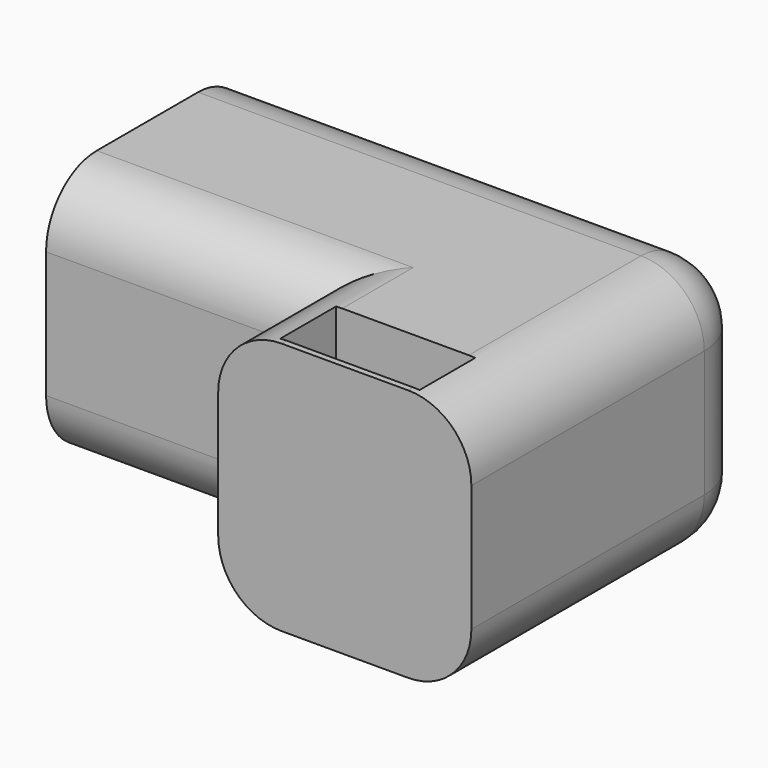
from build123d import *

# Parameters (mm, degrees)
F1_DEPTH     = 20
F2_DEPTH     = 5
F3_R         = 6.25
F4_DEPTH     = 10
F5_R         = 1.4
F6_DEPTH     = 3.9098179487
F7_T1_DEPTH  = 47.5
F7_T3_DEPTH  = 32.5
F7_T5_DEPTH  = 20.5
F7_T7_DEPTH  = 35.5
F7_T9_DEPTH  = 10
F7_S13_W     = 5
F7_S13_H     = 5
F7_T14_DEPTH = 5
F7_S19_W     = 5
F7_S19_H     = 5
F7_T20_DEPTH = 5
F7_T27_DEPTH = 45
F7_T31_DEPTH = 33
F7_T38_DEPTH = 45
F7_T42_DEPTH = 33


# Not quite as in the source:
# - a fillet or chamfer that OpenCascade refuses, or shapes differently, is made with other operations: its cross-section is extruded or revolved along the edge and cut away or added


with BuildPart() as f1:
    # F0 (on Top) → F1 (new body)
    with BuildSketch(Plane.XY):
        Polygon((0, 10), (0, 0), (0, -10), (20, -10), (20, -18), (40, -18), (40, 10), align=None)
        Polygon((35.5, -12), (35.5, -17.5), (30, -17.5), (24.5, -17.5), (24.5, -12), align=None, mode=Mode.SUBTRACT)
    extrude(amount=F1_DEPTH)

    # F0 (on Top) → F2 (join)
    with BuildSketch(Plane.XY):
        Polygon((30, -17.5), (35.5, -17.5), (35.5, -12), (24.5, -12), (24.5, -17.5), align=None)
    extrude(amount=F2_DEPTH)

    # F3 (on face) → F4 (cut)
    with BuildSketch(Plane(origin=(0, 0, 0), x_dir=(0, -1, 0), z_dir=(-1, 0, 0))):
        with Locations((0, 10)):
            Circle(F3_R)
    extrude(amount=-F4_DEPTH, mode=Mode.SUBTRACT)

    # F5 (on face) → F6 (cut, through all)
    with BuildSketch(Plane(origin=(0, 10, 0), x_dir=(-1, 0, 0), z_dir=(0, 1, 0))):
        with Locations((-5, 10)):
            Circle(F5_R)
    extrude(amount=-F6_DEPTH, mode=Mode.SUBTRACT)

    # F7: fillet of radius 5 on 9 edges, made by hand

    # F7_s2 → F7_t1 (cut)
    with BuildSketch(Plane.YZ.offset(-12.5)):
        with BuildLine():
            ThreePointArc((10, 15), (8.5355339059, 18.5355339059), (5, 20))
            Line((5, 20), (10, 20))
            Line((10, 20), (10, 15))
        make_face()
        with BuildLine():
            ThreePointArc((10, 5), (8.5355339059, 1.4644660941), (5, 0))
            Line((5, 0), (10, 0))
            Line((10, 0), (10, 5))
        make_face()
    extrude(amount=F7_T1_DEPTH, mode=Mode.SUBTRACT)

    # F7_s4 → F7_t3 (cut)
    with BuildSketch(Plane.YZ.offset(-12.5)):
        with BuildLine():
            ThreePointArc((-5, 20), (-8.5355339059, 18.5355339059), (-10, 15))
            Line((-10, 15), (-10, 20))
            Line((-10, 20), (-5, 20))
        make_face()
        with BuildLine():
            ThreePointArc((-5, 0), (-8.5355339059, 1.4644660941), (-10, 5))
            Line((-10, 5), (-10, 0))
            Line((-10, 0), (-5, 0))
        make_face()
    extrude(amount=F7_T3_DEPTH, mode=Mode.SUBTRACT)

    # F7_s6 → F7_t5 (cut)
    with BuildSketch(Plane.XZ.offset(10)):
        with BuildLine():
            ThreePointArc((25, 20), (21.4644660941, 18.5355339059), (20, 15))
            Line((20, 15), (20, 20))
            Line((20, 20), (25, 20))
        make_face()
        with BuildLine():
            ThreePointArc((25, 0), (21.4644660941, 1.4644660941), (20, 5))
            Line((20, 5), (20, 0))
            Line((20, 0), (25, 0))
        make_face()
    extrude(amount=F7_T5_DEPTH, mode=Mode.SUBTRACT)

    # F7_s8 → F7_t7 (cut)
    with BuildSketch(Plane.XZ.offset(-5)):
        with BuildLine():
            ThreePointArc((35, 20), (38.5355339059, 18.5355339059), (40, 15))
            Line((40, 15), (40, 20))
            Line((40, 20), (35, 20))
        make_face()
        with BuildLine():
            ThreePointArc((35, 0), (38.5355339059, 1.4644660941), (40, 5))
            Line((40, 5), (40, 0))
            Line((40, 0), (35, 0))
        make_face()
    extrude(amount=F7_T7_DEPTH, mode=Mode.SUBTRACT)

    # F7_s10 → F7_t9 (cut)
    with BuildSketch(Plane.XY.offset(5)):
        with BuildLine():
            ThreePointArc((35, 10), (38.5355339059, 8.5355339059), (40, 5))
            Line((40, 5), (40, 10))
            Line((40, 10), (35, 10))
        make_face()
    extrude(amount=F7_T9_DEPTH, mode=Mode.SUBTRACT)


with BuildPart() as f7_tool12:
    # F7_s13 → F7_t14 (new body)
    with BuildSketch(Plane.XZ.offset(-5)):
        with Locations((37.5, 17.5)):
            Rectangle(F7_S13_W, F7_S13_H)
    extrude(amount=-F7_T14_DEPTH)

    # F7_s15 → F7_t16 (revolve, cut)
    with BuildSketch(Plane(origin=(35, 5, 15), x_dir=(-0.7071067812, 0, -0.7071067812), z_dir=(0.7071067812, 0, -0.7071067812))):
        with BuildLine():
            ThreePointArc((0, -5), (5, 0), (0, 5))
            Line((0, 5), (0, -5))
        make_face()
    revolve(axis=Axis((35, 5, 15), (0, 1, 0)), mode=Mode.SUBTRACT)


with BuildPart() as f1_1:
    add(f1.part)

    # F7_t11: cut F7_tool12
    add(f7_tool12.part, mode=Mode.SUBTRACT)


with BuildPart() as f7_tool18:
    # F7_s19 → F7_t20 (new body)
    with BuildSketch(Plane.XZ.offset(-5)):
        with Locations((37.5, 2.5)):
            Rectangle(F7_S19_W, F7_S19_H)
    extrude(amount=-F7_T20_DEPTH)

    # F7_s21 → F7_t22 (revolve, cut)
    with BuildSketch(Plane(origin=(35, 5, 5), x_dir=(-0.7071067812, 0, 0.7071067812), z_dir=(-0.7071067812, 0, -0.7071067812))):
        with BuildLine():
            ThreePointArc((0, -5), (5, 0), (0, 5))
            Line((0, 5), (0, -5))
        make_face()
    revolve(axis=Axis((35, 5, 5), (0, 1, 0)), mode=Mode.SUBTRACT)


with BuildPart() as f1_2:
    add(f1_1.part)

    # F7_t17: cut F7_tool18
    add(f7_tool18.part, mode=Mode.SUBTRACT)


with BuildPart() as f7_tool25:
    # F7_s26 → F7_t27 (new body)
    with BuildSketch(Plane.YZ.offset(-12.5)):
        with BuildLine():
            ThreePointArc((-5, 20), (-8.5355339059, 18.5355339059), (-10, 15))
            Line((-10, 15), (-10, 20))
            Line((-10, 20), (-5, 20))
        make_face()
    extrude(amount=F7_T27_DEPTH)

    split(bisect_by=Plane.YZ.offset(20), keep=Keep.TOP)


with BuildPart() as f7_tool29:
    # F7_s30 → F7_t31 (new body)
    with BuildSketch(Plane.XZ.offset(-2.5)):
        with BuildLine():
            ThreePointArc((25, 20), (21.4644660941, 18.5355339059), (20, 15))
            Line((20, 15), (20, 20))
            Line((20, 20), (25, 20))
        make_face()
    extrude(amount=F7_T31_DEPTH)

    split(bisect_by=Plane.XZ.offset(10), keep=Keep.BOTTOM)


with BuildPart() as f7_tool25_1:
    add(f7_tool25.part)

    # F7_t33: intersect F7_tool29
    add(f7_tool29.part, mode=Mode.INTERSECT)


with BuildPart() as f1_3:
    add(f1_2.part)

    # F7_t23: cut F7_tool25
    add(f7_tool25_1.part, mode=Mode.SUBTRACT)


with BuildPart() as f7_tool36:
    # F7_s37 → F7_t38 (new body)
    with BuildSketch(Plane.YZ.offset(-12.5)):
        with BuildLine():
            ThreePointArc((-5, 0), (-8.5355339059, 1.4644660941), (-10, 5))
            Line((-10, 5), (-10, 0))
            Line((-10, 0), (-5, 0))
        make_face()
    extrude(amount=F7_T38_DEPTH)

    split(bisect_by=Plane.YZ.offset(20), keep=Keep.TOP)


with BuildPart() as f7_tool40:
    # F7_s41 → F7_t42 (new body)
    with BuildSketch(Plane.XZ.offset(-2.5)):
        with BuildLine():
            ThreePointArc((25, 0), (21.4644660941, 1.4644660941), (20, 5))
            Line((20, 5), (20, 0))
            Line((20, 0), (25, 0))
        make_face()
    extrude(amount=F7_T42_DEPTH)

    split(bisect_by=Plane.XZ.offset(10), keep=Keep.BOTTOM)


with BuildPart() as f7_tool36_1:
    add(f7_tool36.part)

    # F7_t44: intersect F7_tool40
    add(f7_tool40.part, mode=Mode.INTERSECT)


with BuildPart() as f1_4:
    add(f1_3.part)

    # F7_t34: cut F7_tool36
    add(f7_tool36_1.part, mode=Mode.SUBTRACT)


solid = f1_4.part
